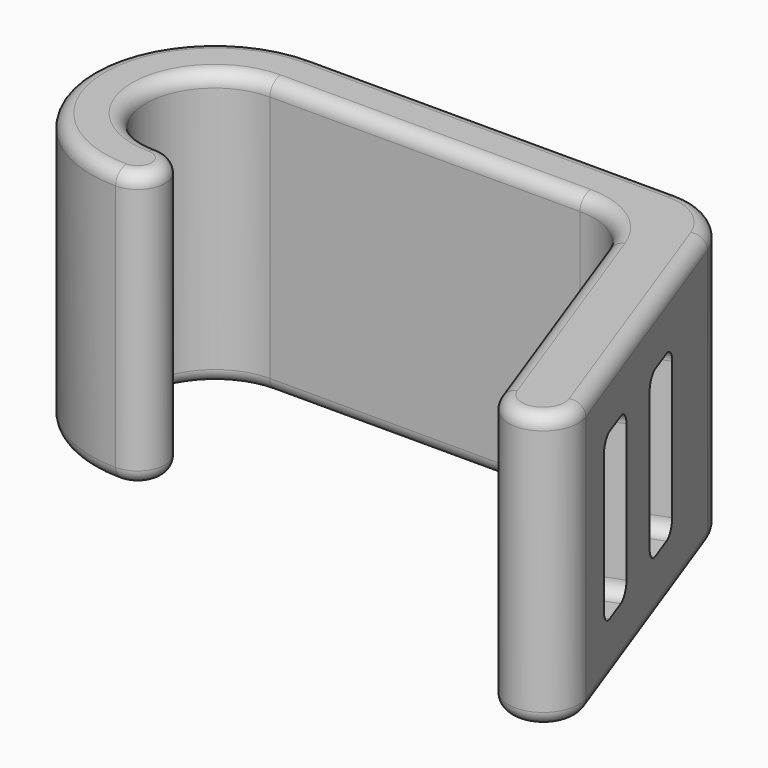
from build123d import *

# Parameters (mm, degrees)
F1_DEPTH    = 20
F3_DEPTH    = 5.1
F4_R        = 5
F5_R        = 1
F6_R        = 1
F7_T1_DEPTH = 20
F7_T4_ANGLE = 70
F7_T6_ANGLE = 70


# Not quite as in the source:
# - a fillet or chamfer that OpenCascade refuses, or shapes differently, is made with other operations: its cross-section is extruded or revolved along the edge and cut away or added


with BuildPart() as f1:
    # F0 (on Top) → F1 (new body)
    with BuildSketch(Plane.XY):
        with BuildLine():
            Line((30, 0), (0, 0))
            ThreePointArc((0, 0), (-9, -9), (0, -18))
            ThreePointArc((0, -18), (2, -16), (0, -14))
            ThreePointArc((0, -14), (-5, -9), (0, -4))
            Line((0, -4), (26.0285742974, -4))
            Line((26.0285742974, -4), (33.7580712171, -25.2366182506))
            ThreePointArc((33.7580712171, -25.2366182506), (37.0264387656, -26.7606830681), (38.5505035831, -23.4923155196))
            Line((38.5505035831, -23.4923155196), (30, 0))
        make_face()
    extrude(amount=F1_DEPTH)

    # F2 (on face) → F3 (cut, through all)
    with BuildSketch(Plane(origin=(26.4906666468, 9.6418141453, 0), x_dir=(-0.3420201433, 0.9396926208, 0), z_dir=(0.9396926208, 0.3420201433, 0))):
        with BuildLine():
            ThreePointArc((-19.9606042998, 15), (-20.2534975186, 15.7071067812), (-20.9606042998, 16))
            Line((-20.9606042998, 16), (-22.9606042998, 16))
            ThreePointArc((-22.9606042998, 16), (-23.667711081, 15.7071067812), (-23.9606042998, 15))
            Line((-23.9606042998, 15), (-23.9606042998, 5))
            ThreePointArc((-23.9606042998, 5), (-23.667711081, 4.2928932188), (-22.9606042998, 4))
            Line((-22.9606042998, 4), (-20.9606042998, 4))
            ThreePointArc((-20.9606042998, 4), (-20.2534975186, 4.2928932188), (-19.9606042998, 5))
            Line((-19.9606042998, 5), (-19.9606042998, 15))
        make_face()
        with BuildLine():
            ThreePointArc((-28.0606042998, 15), (-28.3534975186, 15.7071067812), (-29.0606042998, 16))
            Line((-29.0606042998, 16), (-31.0606042998, 16))
            ThreePointArc((-31.0606042998, 16), (-31.767711081, 15.7071067812), (-32.0606042998, 15))
            Line((-32.0606042998, 15), (-32.0606042998, 5))
            ThreePointArc((-32.0606042998, 5), (-31.767711081, 4.2928932188), (-31.0606042998, 4))
            Line((-31.0606042998, 4), (-29.0606042998, 4))
            ThreePointArc((-29.0606042998, 4), (-28.3534975186, 4.2928932188), (-28.0606042998, 5))
            Line((-28.0606042998, 5), (-28.0606042998, 15))
        make_face()
    extrude(amount=-F3_DEPTH, mode=Mode.SUBTRACT)

    # F4
    f4_edges = [f1.edges().sort_by_distance(p)[0] for p in [
        (26.028574, -4, 10),
    ]]
    fillet(f4_edges, radius=F4_R)

    # F5
    f5_edges = [f1.edges().sort_by_distance(p)[0] for p in [
        (15, 0, 20),
        (11.263768, -4, 20),
        (25.395419, -4.90424, 20),
        (-5, -9, 20),
        (30.492035, -16.263259, 20),
        (2, -16, 20),
        (37.026439, -26.760683, 20),
        (-9, -9, 20),
        (34.275252, -11.746158, 20),
    ]]
    fillet(f5_edges, radius=F5_R)

    # F6
    f6_edges = [f1.edges().sort_by_distance(p)[0] for p in [
        (11.263768, -4, 0),
        (25.395419, -4.90424, 0),
        (-5, -9, 0),
        (30.492035, -16.263259, 0),
        (2, -16, 0),
        (37.026439, -26.760683, 0),
        (-9, -9, 0),
        (34.275252, -11.746158, 0),
        (15, 0, 0),
    ]]
    fillet(f6_edges, radius=F6_R)

    # F7: fillet of radius 5 on 1 edges, made by hand

    # F7_s2 → F7_t1 (cut)
    with BuildSketch(Plane.XY):
        with BuildLine():
            ThreePointArc((31.1982351897, -3.290954605), (29.3668444907, -0.9042397786), (26.497693671, 0.0004))
            Line((26.497693671, 0.0004), (26.497693671, 0.5006211803))
            ThreePointArc((26.497693671, 0.5006211803), (28.2488468355, 0.5002211803), (30, 0.5002211803))
            Line((30, 0.5002211803), (30.4700541519, 0.1710857198))
            ThreePointArc((30.4700541519, 0.1710857198), (31.0689838082, -1.4744599868), (31.6682893415, -3.1198688852))
            Line((31.6682893415, -3.1198688852), (31.1982351897, -3.290954605))
        make_face()
    extrude(amount=F7_T1_DEPTH, mode=Mode.SUBTRACT)

    # F7_s3 → F7_t4 (revolve, cut)
    with BuildSketch(Plane.YZ.offset(26.497693671)):
        with BuildLine():
            ThreePointArc((-0.9996, 0), (-0.2924932188, 0.2928932188), (0.0004, 1))
            Line((0.0004, 1), (0.0004, 0))
            Line((0.0004, 0), (-0.9996, 0))
        make_face()
    revolve(axis=Axis((26.497693671, -5.0018118027, 0), (0, 0, -1)), revolution_arc=F7_T4_ANGLE, mode=Mode.SUBTRACT)

    # F7_s5 → F7_t6 (revolve, cut)
    with BuildSketch(Plane(origin=(4.7071926658, -12.9329055584, 0), x_dir=(0, 0, 1), z_dir=(0.3420201433, -0.9396926208, 0))):
        with BuildLine():
            ThreePointArc((20, -27.1911786236), (19.7071067812, -27.8982854048), (19, -28.1911786236))
            Line((19, -28.1911786236), (20, -28.1911786236))
            Line((20, -28.1911786236), (20, -27.1911786236))
        make_face()
    revolve(axis=Axis((26.497693671, -5.0018118027, 20), (0, 0, 1)), revolution_arc=F7_T6_ANGLE, mode=Mode.SUBTRACT)


solid = f1.part
